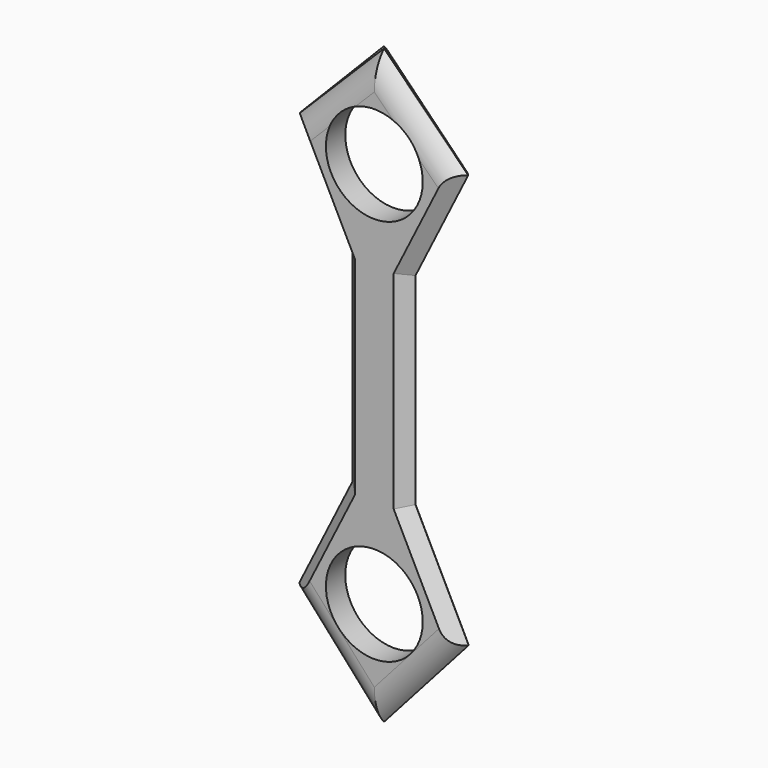
from build123d import *

# Parameters (mm, degrees)
F0_R          = 6.35
F1_DEPTH      = 1.5875
F2_R          = 6.35
F3_DEPTH      = 1.5875
F4_T4_DEPTH   = 44.9962243683
F4_T10_DEPTH  = 44.9962243683
F4_T16_DEPTH  = 44.9962243683
F4_T22_DEPTH  = 44.9962243683
F4_T28_DEPTH  = 33.7952560254
F4_T33_DEPTH  = 33.7952560254
F4_T38_DEPTH  = 33.7952560254
F4_T43_DEPTH  = 33.7952560254
F4_T48_DEPTH  = 33.7952560254
F4_T53_DEPTH  = 33.7952560254
F4_T58_DEPTH  = 33.7952560254
F4_T63_DEPTH  = 33.7952560254
F4_T69_DEPTH  = 44.9962243683
F4_T73_DEPTH  = 33.7952560254
F4_T80_DEPTH  = 33.7952560254
F4_T84_DEPTH  = 44.9962243683
F4_T91_DEPTH  = 33.7952560254
F4_T95_DEPTH  = 44.9962243683
F4_T102_DEPTH = 44.9962243683
F4_T106_DEPTH = 33.7952560254
F4_T113_DEPTH = 33.7952560254
F4_T117_DEPTH = 44.9962243683
F4_T124_DEPTH = 44.9962243683
F4_T128_DEPTH = 33.7952560254
F4_T135_DEPTH = 33.7952560254
F4_T139_DEPTH = 44.9962243683
F4_T146_DEPTH = 44.9962243683
F4_T150_DEPTH = 33.7952560254
F5_T1_DEPTH   = 30.2674508006
F5_T3_DEPTH   = 30.4563843948
F5_T5_DEPTH   = 30.4563843948
F5_T7_DEPTH   = 30.2674508006
F5_T9_DEPTH   = 29.4174556361
F5_T11_DEPTH  = 29.6012389831
F5_T13_DEPTH  = 29.6012389831
F5_T15_DEPTH  = 29.4174556361


# Not quite as in the source:
# - a fillet or chamfer that OpenCascade refuses, or shapes differently, is made with other operations: its cross-section is extruded or revolved along the edge and cut away or added


with BuildPart() as f1:
    # F0 (on Front) → F1 (new body)
    with BuildSketch(Plane.XZ):
        Polygon((-12.7, 0), (0, -14.245194383), (12.7, 0), (6.35, 12.7), (6.35, 25.4), (6.35, 38.1), (12.7, 50.8), (0, 63.5), (-12.7, 50.8), (-6.35, 38.1), (-6.35, 12.7), align=None)
        Circle(F0_R, mode=Mode.SUBTRACT)
        with Locations((0, 50.8)):
            Circle(F0_R, mode=Mode.SUBTRACT)
    extrude(amount=F1_DEPTH)

    # F2 (on Front) → F3 (join)
    with BuildSketch(Plane.XZ):
        Polygon((0, -13.97), (12.7, 0), (6.35, 12.7), (6.35, 25.4), (6.35, 38.1), (12.7, 50.8), (0, 63.7794), (-12.7, 50.8), (-6.35, 38.1), (-6.35, 25.4), (-6.35, 12.7), (-12.7, 0), align=None)
        Circle(F2_R, mode=Mode.SUBTRACT)
        with Locations((0, 50.8)):
            Circle(F2_R, mode=Mode.SUBTRACT)
    extrude(amount=-F3_DEPTH)

    # F4: chamfer of 3.81 on 12 edges, made by hand


with BuildPart() as f4_tool2:
    # F4_s3 → F4_t4 (new body)
    with BuildSketch(Plane.XY.offset(47.8981121842)):
        Polygon((2.54, -1.5875), (6.35, 2.2225), (6.35, -1.5875), align=None)
    extrude(amount=-F4_T4_DEPTH)

    split(bisect_by=Plane(origin=(-10.16, 0, 5.08), x_dir=(0, 1, 0), z_dir=(0.894427191, 0, -0.4472135955)), keep=Keep.TOP)

    split(bisect_by=Plane(origin=(10.16, 0, 5.08), x_dir=(0, 1, 0), z_dir=(0.894427191, 0, 0.4472135955)), keep=Keep.TOP)


with BuildPart() as f1_1:
    add(f1.part)

    # F4_t1: cut F4_tool2
    add(f4_tool2.part, mode=Mode.SUBTRACT)


with BuildPart() as f4_tool8:
    # F4_s9 → F4_t10 (new body)
    with BuildSketch(Plane.XY.offset(2.9018878158)):
        Polygon((2.54, 1.5875), (6.35, -2.2225), (6.35, 1.5875), align=None)
    extrude(amount=F4_T10_DEPTH)

    split(bisect_by=Plane(origin=(-10.16, 0, 5.08), x_dir=(0, 1, 0), z_dir=(0.894427191, 0, -0.4472135955)), keep=Keep.TOP)

    split(bisect_by=Plane(origin=(10.16, 0, 5.08), x_dir=(0, 1, 0), z_dir=(0.894427191, 0, 0.4472135955)), keep=Keep.TOP)


with BuildPart() as f1_2:
    add(f1_1.part)

    # F4_t7: cut F4_tool8
    add(f4_tool8.part, mode=Mode.SUBTRACT)


with BuildPart() as f4_tool14:
    # F4_s15 → F4_t16 (new body)
    with BuildSketch(Plane.XY.offset(47.8981121842)):
        Polygon((-2.54, 1.5875), (-6.35, -2.2225), (-6.35, 1.5875), align=None)
    extrude(amount=-F4_T16_DEPTH)

    split(bisect_by=Plane(origin=(10.16, 0, 5.08), x_dir=(0, 1, 0), z_dir=(-0.894427191, 0, -0.4472135955)), keep=Keep.TOP)

    split(bisect_by=Plane(origin=(-10.16, 0, 5.08), x_dir=(0, 1, 0), z_dir=(-0.894427191, 0, 0.4472135955)), keep=Keep.TOP)


with BuildPart() as f1_3:
    add(f1_2.part)

    # F4_t13: cut F4_tool14
    add(f4_tool14.part, mode=Mode.SUBTRACT)


with BuildPart() as f4_tool20:
    # F4_s21 → F4_t22 (new body)
    with BuildSketch(Plane.XY.offset(47.8981121842)):
        Polygon((-2.54, -1.5875), (-6.35, 2.2225), (-6.35, -1.5875), align=None)
    extrude(amount=-F4_T22_DEPTH)

    split(bisect_by=Plane(origin=(10.16, 0, 5.08), x_dir=(0, 1, 0), z_dir=(-0.894427191, 0, -0.4472135955)), keep=Keep.TOP)

    split(bisect_by=Plane(origin=(-10.16, 0, 5.08), x_dir=(0, 1, 0), z_dir=(-0.894427191, 0, 0.4472135955)), keep=Keep.TOP)


with BuildPart() as f1_4:
    add(f1_3.part)

    # F4_t19: cut F4_tool20
    add(f4_tool20.part, mode=Mode.SUBTRACT)


with BuildPart() as f4_tool26:
    # F4_s27 → F4_t28 (new body)
    with BuildSketch(Plane(origin=(12.128151021, 0, 24.256302042), x_dir=(0, 1, 0), z_dir=(0.4472135955, 0, 0.894427191))):
        Polygon((-1.5875, 15.1692253257), (2.2225, 11.3592253257), (-1.5875, 11.3592253257), align=None)
    extrude(amount=F4_T28_DEPTH)

    split(bisect_by=Plane.YZ.offset(6.35), keep=Keep.TOP)


with BuildPart() as f1_5:
    add(f1_4.part)

    # F4_t25: cut F4_tool26
    add(f4_tool26.part, mode=Mode.SUBTRACT)


with BuildPart() as f4_tool31:
    # F4_s32 → F4_t33 (new body)
    with BuildSketch(Plane(origin=(-27.241848979, 0, 54.483697958), x_dir=(0, 1, 0), z_dir=(0.4472135955, 0, -0.894427191))):
        Polygon((-1.5875, 15.1692253257), (2.2225, 11.3592253257), (-1.5875, 11.3592253257), align=None)
    extrude(amount=F4_T33_DEPTH)

    split(bisect_by=Plane.YZ.offset(-6.35), keep=Keep.BOTTOM)


with BuildPart() as f1_6:
    add(f1_5.part)

    # F4_t30: cut F4_tool31
    add(f4_tool31.part, mode=Mode.SUBTRACT)


with BuildPart() as f4_tool36:
    # F4_s37 → F4_t38 (new body)
    with BuildSketch(Plane(origin=(6.921848979, 0, -13.843697958), x_dir=(0, 1, 0), z_dir=(-0.4472135955, 0, 0.894427191))):
        Polygon((-1.5875, -7.5492253257), (2.2225, -11.3592253257), (-1.5875, -11.3592253257), align=None)
    extrude(amount=F4_T38_DEPTH)

    split(bisect_by=Plane.YZ.offset(6.35), keep=Keep.TOP)


with BuildPart() as f1_7:
    add(f1_6.part)

    # F4_t35: cut F4_tool36
    add(f4_tool36.part, mode=Mode.SUBTRACT)


with BuildPart() as f4_tool41:
    # F4_s42 → F4_t43 (new body)
    with BuildSketch(Plane(origin=(8.191848979, 0, 16.383697958), x_dir=(0, 1, 0), z_dir=(-0.4472135955, 0, -0.894427191))):
        Polygon((-1.5875, -7.5492253257), (2.2225, -11.3592253257), (-1.5875, -11.3592253257), align=None)
    extrude(amount=F4_T43_DEPTH)

    split(bisect_by=Plane.YZ.offset(-6.35), keep=Keep.BOTTOM)


with BuildPart() as f1_8:
    add(f1_7.part)

    # F4_t40: cut F4_tool41
    add(f4_tool41.part, mode=Mode.SUBTRACT)


with BuildPart() as f4_tool46:
    # F4_s47 → F4_t48 (new body)
    with BuildSketch(Plane(origin=(8.191848979, 0, 16.383697958), x_dir=(0, 1, 0), z_dir=(-0.4472135955, 0, -0.894427191))):
        Polygon((1.5875, -7.5492253257), (-2.2225, -11.3592253257), (1.5875, -11.3592253257), align=None)
    extrude(amount=F4_T48_DEPTH)

    split(bisect_by=Plane.YZ.offset(-6.35), keep=Keep.BOTTOM)


with BuildPart() as f1_9:
    add(f1_8.part)

    # F4_t45: cut F4_tool46
    add(f4_tool46.part, mode=Mode.SUBTRACT)


with BuildPart() as f4_tool51:
    # F4_s52 → F4_t53 (new body)
    with BuildSketch(Plane(origin=(6.921848979, 0, -13.843697958), x_dir=(0, 1, 0), z_dir=(-0.4472135955, 0, 0.894427191))):
        Polygon((1.5875, -7.5492253257), (-2.2225, -11.3592253257), (1.5875, -11.3592253257), align=None)
    extrude(amount=F4_T53_DEPTH)

    split(bisect_by=Plane.YZ.offset(6.35), keep=Keep.TOP)


with BuildPart() as f1_10:
    add(f1_9.part)

    # F4_t50: cut F4_tool51
    add(f4_tool51.part, mode=Mode.SUBTRACT)


with BuildPart() as f4_tool56:
    # F4_s57 → F4_t58 (new body)
    with BuildSketch(Plane(origin=(-27.241848979, 0, 54.483697958), x_dir=(0, 1, 0), z_dir=(0.4472135955, 0, -0.894427191))):
        Polygon((1.5875, 15.1692253257), (-2.2225, 11.3592253257), (1.5875, 11.3592253257), align=None)
    extrude(amount=F4_T58_DEPTH)

    split(bisect_by=Plane.YZ.offset(-6.35), keep=Keep.BOTTOM)


with BuildPart() as f1_11:
    add(f1_10.part)

    # F4_t55: cut F4_tool56
    add(f4_tool56.part, mode=Mode.SUBTRACT)


with BuildPart() as f4_tool61:
    # F4_s62 → F4_t63 (new body)
    with BuildSketch(Plane(origin=(12.128151021, 0, 24.256302042), x_dir=(0, 1, 0), z_dir=(0.4472135955, 0, 0.894427191))):
        Polygon((1.5875, 15.1692253257), (-2.2225, 11.3592253257), (1.5875, 11.3592253257), align=None)
    extrude(amount=F4_T63_DEPTH)

    split(bisect_by=Plane.YZ.offset(6.35), keep=Keep.TOP)


with BuildPart() as f1_12:
    add(f1_11.part)

    # F4_t60: cut F4_tool61
    add(f4_tool61.part, mode=Mode.SUBTRACT)


with BuildPart() as f4_tool67:
    # F4_s68 → F4_t69 (new body)
    with BuildSketch(Plane.XY.offset(47.8981121842)):
        Polygon((2.54, -1.5875), (6.35, 2.2225), (6.35, -1.5875), align=None)
    extrude(amount=-F4_T69_DEPTH)

    split(bisect_by=Plane(origin=(-10.16, 0, 5.08), x_dir=(0, 1, 0), z_dir=(-0.894427191, 0, 0.4472135955)), keep=Keep.TOP)


with BuildPart() as f4_tool71:
    # F4_s72 → F4_t73 (new body)
    with BuildSketch(Plane(origin=(12.128151021, 0, 24.256302042), x_dir=(0, 1, 0), z_dir=(0.4472135955, 0, 0.894427191))):
        Polygon((-1.5875, 15.1692253257), (2.2225, 11.3592253257), (-1.5875, 11.3592253257), align=None)
    extrude(amount=F4_T73_DEPTH)

    split(bisect_by=Plane.YZ.offset(6.35), keep=Keep.BOTTOM)


with BuildPart() as f4_tool67_1:
    add(f4_tool67.part)

    # F4_t75: intersect F4_tool71
    add(f4_tool71.part, mode=Mode.INTERSECT)


with BuildPart() as f1_13:
    add(f1_12.part)

    # F4_t65: cut F4_tool67
    add(f4_tool67_1.part, mode=Mode.SUBTRACT)


with BuildPart() as f4_tool78:
    # F4_s79 → F4_t80 (new body)
    with BuildSketch(Plane(origin=(6.921848979, 0, -13.843697958), x_dir=(0, 1, 0), z_dir=(-0.4472135955, 0, 0.894427191))):
        Polygon((-1.5875, -7.5492253257), (2.2225, -11.3592253257), (-1.5875, -11.3592253257), align=None)
    extrude(amount=F4_T80_DEPTH)

    split(bisect_by=Plane.YZ.offset(6.35), keep=Keep.BOTTOM)


with BuildPart() as f4_tool82:
    # F4_s83 → F4_t84 (new body)
    with BuildSketch(Plane.XY.offset(47.8981121842)):
        Polygon((2.54, -1.5875), (6.35, 2.2225), (6.35, -1.5875), align=None)
    extrude(amount=-F4_T84_DEPTH)

    split(bisect_by=Plane(origin=(10.16, 0, 5.08), x_dir=(0, 1, 0), z_dir=(-0.894427191, 0, -0.4472135955)), keep=Keep.TOP)


with BuildPart() as f4_tool78_1:
    add(f4_tool78.part)

    # F4_t86: intersect F4_tool82
    add(f4_tool82.part, mode=Mode.INTERSECT)


with BuildPart() as f1_14:
    add(f1_13.part)

    # F4_t76: cut F4_tool78
    add(f4_tool78_1.part, mode=Mode.SUBTRACT)


with BuildPart() as f4_tool89:
    # F4_s90 → F4_t91 (new body)
    with BuildSketch(Plane(origin=(6.921848979, 0, -13.843697958), x_dir=(0, 1, 0), z_dir=(-0.4472135955, 0, 0.894427191))):
        Polygon((1.5875, -7.5492253257), (-2.2225, -11.3592253257), (1.5875, -11.3592253257), align=None)
    extrude(amount=F4_T91_DEPTH)

    split(bisect_by=Plane.YZ.offset(6.35), keep=Keep.BOTTOM)


with BuildPart() as f4_tool93:
    # F4_s94 → F4_t95 (new body)
    with BuildSketch(Plane.XY.offset(2.9018878158)):
        Polygon((2.54, 1.5875), (6.35, -2.2225), (6.35, 1.5875), align=None)
    extrude(amount=F4_T95_DEPTH)

    split(bisect_by=Plane(origin=(10.16, 0, 5.08), x_dir=(0, 1, 0), z_dir=(-0.894427191, 0, -0.4472135955)), keep=Keep.TOP)


with BuildPart() as f4_tool89_1:
    add(f4_tool89.part)

    # F4_t97: intersect F4_tool93
    add(f4_tool93.part, mode=Mode.INTERSECT)


with BuildPart() as f1_15:
    add(f1_14.part)

    # F4_t87: cut F4_tool89
    add(f4_tool89_1.part, mode=Mode.SUBTRACT)


with BuildPart() as f4_tool100:
    # F4_s101 → F4_t102 (new body)
    with BuildSketch(Plane.XY.offset(2.9018878158)):
        Polygon((2.54, 1.5875), (6.35, -2.2225), (6.35, 1.5875), align=None)
    extrude(amount=F4_T102_DEPTH)

    split(bisect_by=Plane(origin=(-10.16, 0, 5.08), x_dir=(0, 1, 0), z_dir=(-0.894427191, 0, 0.4472135955)), keep=Keep.TOP)


with BuildPart() as f4_tool104:
    # F4_s105 → F4_t106 (new body)
    with BuildSketch(Plane(origin=(12.128151021, 0, 24.256302042), x_dir=(0, 1, 0), z_dir=(0.4472135955, 0, 0.894427191))):
        Polygon((1.5875, 15.1692253257), (-2.2225, 11.3592253257), (1.5875, 11.3592253257), align=None)
    extrude(amount=F4_T106_DEPTH)

    split(bisect_by=Plane.YZ.offset(6.35), keep=Keep.BOTTOM)


with BuildPart() as f4_tool100_1:
    add(f4_tool100.part)

    # F4_t108: intersect F4_tool104
    add(f4_tool104.part, mode=Mode.INTERSECT)


with BuildPart() as f1_16:
    add(f1_15.part)

    # F4_t98: cut F4_tool100
    add(f4_tool100_1.part, mode=Mode.SUBTRACT)


with BuildPart() as f4_tool111:
    # F4_s112 → F4_t113 (new body)
    with BuildSketch(Plane(origin=(-27.241848979, 0, 54.483697958), x_dir=(0, 1, 0), z_dir=(0.4472135955, 0, -0.894427191))):
        Polygon((1.5875, 15.1692253257), (-2.2225, 11.3592253257), (1.5875, 11.3592253257), align=None)
    extrude(amount=F4_T113_DEPTH)

    split(bisect_by=Plane.YZ.offset(-6.35), keep=Keep.TOP)


with BuildPart() as f4_tool115:
    # F4_s116 → F4_t117 (new body)
    with BuildSketch(Plane.XY.offset(47.8981121842)):
        Polygon((-2.54, 1.5875), (-6.35, -2.2225), (-6.35, 1.5875), align=None)
    extrude(amount=-F4_T117_DEPTH)

    split(bisect_by=Plane(origin=(10.16, 0, 5.08), x_dir=(0, 1, 0), z_dir=(0.894427191, 0, 0.4472135955)), keep=Keep.TOP)


with BuildPart() as f4_tool111_1:
    add(f4_tool111.part)

    # F4_t119: intersect F4_tool115
    add(f4_tool115.part, mode=Mode.INTERSECT)


with BuildPart() as f1_17:
    add(f1_16.part)

    # F4_t109: cut F4_tool111
    add(f4_tool111_1.part, mode=Mode.SUBTRACT)


with BuildPart() as f4_tool122:
    # F4_s123 → F4_t124 (new body)
    with BuildSketch(Plane.XY.offset(47.8981121842)):
        Polygon((-2.54, 1.5875), (-6.35, -2.2225), (-6.35, 1.5875), align=None)
    extrude(amount=-F4_T124_DEPTH)

    split(bisect_by=Plane(origin=(-10.16, 0, 5.08), x_dir=(0, 1, 0), z_dir=(0.894427191, 0, -0.4472135955)), keep=Keep.TOP)


with BuildPart() as f4_tool126:
    # F4_s127 → F4_t128 (new body)
    with BuildSketch(Plane(origin=(8.191848979, 0, 16.383697958), x_dir=(0, 1, 0), z_dir=(-0.4472135955, 0, -0.894427191))):
        Polygon((1.5875, -7.5492253257), (-2.2225, -11.3592253257), (1.5875, -11.3592253257), align=None)
    extrude(amount=F4_T128_DEPTH)

    split(bisect_by=Plane.YZ.offset(-6.35), keep=Keep.TOP)


with BuildPart() as f4_tool122_1:
    add(f4_tool122.part)

    # F4_t130: intersect F4_tool126
    add(f4_tool126.part, mode=Mode.INTERSECT)


with BuildPart() as f1_18:
    add(f1_17.part)

    # F4_t120: cut F4_tool122
    add(f4_tool122_1.part, mode=Mode.SUBTRACT)


with BuildPart() as f4_tool133:
    # F4_s134 → F4_t135 (new body)
    with BuildSketch(Plane(origin=(-27.241848979, 0, 54.483697958), x_dir=(0, 1, 0), z_dir=(0.4472135955, 0, -0.894427191))):
        Polygon((-1.5875, 15.1692253257), (2.2225, 11.3592253257), (-1.5875, 11.3592253257), align=None)
    extrude(amount=F4_T135_DEPTH)

    split(bisect_by=Plane.YZ.offset(-6.35), keep=Keep.TOP)


with BuildPart() as f4_tool137:
    # F4_s138 → F4_t139 (new body)
    with BuildSketch(Plane.XY.offset(47.8981121842)):
        Polygon((-2.54, -1.5875), (-6.35, 2.2225), (-6.35, -1.5875), align=None)
    extrude(amount=-F4_T139_DEPTH)

    split(bisect_by=Plane(origin=(10.16, 0, 5.08), x_dir=(0, 1, 0), z_dir=(0.894427191, 0, 0.4472135955)), keep=Keep.TOP)


with BuildPart() as f4_tool133_1:
    add(f4_tool133.part)

    # F4_t141: intersect F4_tool137
    add(f4_tool137.part, mode=Mode.INTERSECT)


with BuildPart() as f1_19:
    add(f1_18.part)

    # F4_t131: cut F4_tool133
    add(f4_tool133_1.part, mode=Mode.SUBTRACT)


with BuildPart() as f4_tool144:
    # F4_s145 → F4_t146 (new body)
    with BuildSketch(Plane.XY.offset(47.8981121842)):
        Polygon((-2.54, -1.5875), (-6.35, 2.2225), (-6.35, -1.5875), align=None)
    extrude(amount=-F4_T146_DEPTH)

    split(bisect_by=Plane(origin=(-10.16, 0, 5.08), x_dir=(0, 1, 0), z_dir=(0.894427191, 0, -0.4472135955)), keep=Keep.TOP)


with BuildPart() as f4_tool148:
    # F4_s149 → F4_t150 (new body)
    with BuildSketch(Plane(origin=(8.191848979, 0, 16.383697958), x_dir=(0, 1, 0), z_dir=(-0.4472135955, 0, -0.894427191))):
        Polygon((-1.5875, -7.5492253257), (2.2225, -11.3592253257), (-1.5875, -11.3592253257), align=None)
    extrude(amount=F4_T150_DEPTH)

    split(bisect_by=Plane.YZ.offset(-6.35), keep=Keep.TOP)


with BuildPart() as f4_tool144_1:
    add(f4_tool144.part)

    # F4_t152: intersect F4_tool148
    add(f4_tool148.part, mode=Mode.INTERSECT)


with BuildPart() as f1_20:
    add(f1_19.part)

    # F4_t142: cut F4_tool144
    add(f4_tool144_1.part, mode=Mode.SUBTRACT)

    # F5: fillet of radius 3.81 on 8 edges, made by hand

    # F5_s2 → F5_t1 (cut)
    with BuildSketch(Plane(origin=(-8.2025518457, 0, 9.0228070302), x_dir=(0, 1, 0), z_dir=(0.672672794, 0, -0.7399400734))):
        with BuildLine():
            ThreePointArc((1.5875, -6.3026317277), (1.167472345, -8.0416508477), (0, -9.3972389321))
            Line((0, -9.3972389321), (1.5875, -9.3972389321))
            Line((1.5875, -9.3972389321), (1.5875, -6.3026317277))
        make_face()
    extrude(amount=F5_T1_DEPTH, mode=Mode.SUBTRACT)

    # F5_s4 → F5_t3 (cut)
    with BuildSketch(Plane(origin=(-12.2242778962, 0, -13.7115917183), x_dir=(0, 1, 0), z_dir=(0.6654638546, 0, 0.7464300759))):
        with BuildLine():
            ThreePointArc((-1.5875, -6.3850547594), (-1.167472345, -8.1240738795), (0, -9.4796619639))
            Line((0, -9.4796619639), (-1.5875, -9.4796619639))
            Line((-1.5875, -9.4796619639), (-1.5875, -6.3850547594))
        make_face()
    extrude(amount=F5_T3_DEPTH, mode=Mode.SUBTRACT)

    # F5_s6 → F5_t5 (cut)
    with BuildSketch(Plane(origin=(-8.0433450609, 0, 9.021969597), x_dir=(0, 1, 0), z_dir=(0.6654638546, 0, -0.7464300759))):
        with BuildLine():
            ThreePointArc((0, -9.4796619639), (-1.167472345, -8.1240738795), (-1.5875, -6.3850547594))
            Line((-1.5875, -6.3850547594), (-1.5875, -9.4796619639))
            Line((-1.5875, -9.4796619639), (0, -9.4796619639))
        make_face()
    extrude(amount=F5_T5_DEPTH, mode=Mode.SUBTRACT)

    # F5_s8 → F5_t7 (cut)
    with BuildSketch(Plane(origin=(-12.1575388515, 0, -13.3732927367), x_dir=(0, 1, 0), z_dir=(0.672672794, 0, 0.7399400734))):
        with BuildLine():
            ThreePointArc((1.5875, -6.3026317277), (1.167472345, -8.0416508477), (0, -9.3972389321))
            Line((0, -9.3972389321), (1.5875, -9.3972389321))
            Line((1.5875, -9.3972389321), (1.5875, -6.3026317277))
        make_face()
    extrude(amount=F5_T7_DEPTH, mode=Mode.SUBTRACT)

    # F5_s10 → F5_t9 (cut)
    with BuildSketch(Plane(origin=(-16.4192619829, 0, 16.4192619829), x_dir=(0, 1, 0), z_dir=(-0.7071067812, 0, 0.7071067812))):
        with BuildLine():
            ThreePointArc((0, -44.9012806053), (-1.167472345, -43.5456925209), (-1.5875, -41.8066734009))
            Line((-1.5875, -41.8066734009), (-1.5875, -44.9012806053))
            Line((-1.5875, -44.9012806053), (0, -44.9012806053))
        make_face()
    extrude(amount=F5_T9_DEPTH, mode=Mode.SUBTRACT)

    # F5_s12 → F5_t11 (cut)
    with BuildSketch(Plane(origin=(-16.590580457, 0, 16.955573227), x_dir=(0, 1, 0), z_dir=(-0.6993718406, 0, 0.714758021))):
        with BuildLine():
            ThreePointArc((1.5875, -41.5109091627), (1.167472345, -43.2499282828), (0, -44.6055163672))
            Line((0, -44.6055163672), (1.5875, -44.6055163672))
            Line((1.5875, -44.6055163672), (1.5875, -41.5109091627))
        make_face()
    extrude(amount=F5_T11_DEPTH, mode=Mode.SUBTRACT)

    # F5_s14 → F5_t13 (cut)
    with BuildSketch(Plane(origin=(37.2928534472, 0, 38.113296223), x_dir=(0, 1, 0), z_dir=(-0.6993718406, 0, -0.714758021))):
        with BuildLine():
            ThreePointArc((1.5875, -41.5109091627), (1.167472345, -43.2499282828), (0, -44.6055163672))
            Line((0, -44.6055163672), (1.5875, -44.6055163672))
            Line((1.5875, -44.6055163672), (1.5875, -41.5109091627))
        make_face()
    extrude(amount=F5_T13_DEPTH, mode=Mode.SUBTRACT)

    # F5_s16 → F5_t15 (cut)
    with BuildSketch(Plane(origin=(37.2205443485, 0, 37.2205443485), x_dir=(0, 1, 0), z_dir=(-0.7071067812, 0, -0.7071067812))):
        with BuildLine():
            ThreePointArc((0, -44.9012806053), (-1.167472345, -43.5456925209), (-1.5875, -41.8066734009))
            Line((-1.5875, -41.8066734009), (-1.5875, -44.9012806053))
            Line((-1.5875, -44.9012806053), (0, -44.9012806053))
        make_face()
    extrude(amount=F5_T15_DEPTH, mode=Mode.SUBTRACT)


solid = f1_20.part
